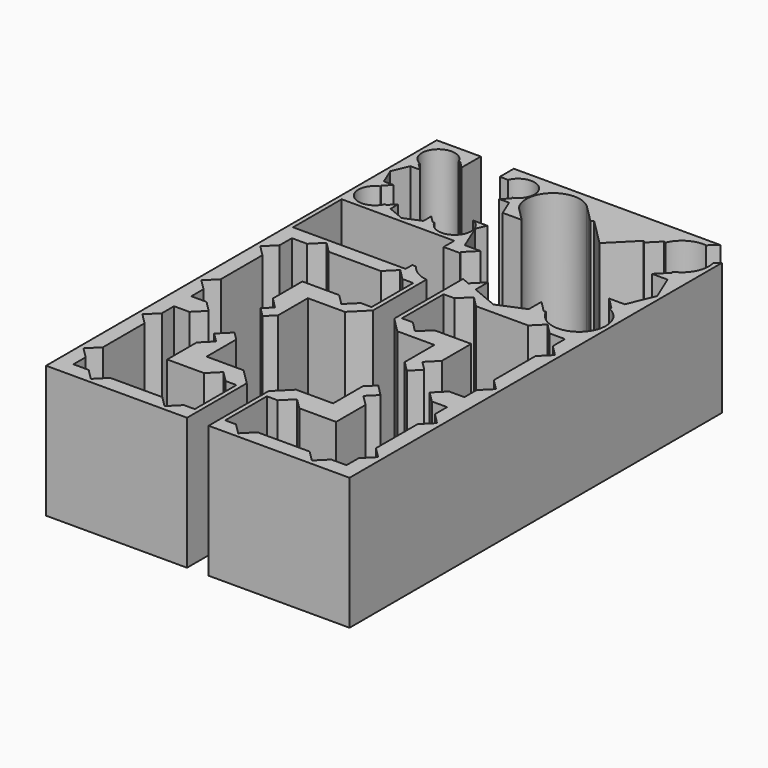
from build123d import *

# Parameters (mm, degrees)
F1_DEPTH = 4499.991


# Not quite as in the source:
# - ends of sketch curves that miss each other by under 0.0002 mm in the source are joined


with BuildPart() as f1:
    # F0 (on Top) → F1 (new body)
    with BuildSketch(Plane.XY):
        with BuildLine():
            Line((11073.483338, 6645.118502), (11073.483338, 4872.327475))
            Line((11073.483338, 4872.327475), (15876.504585, 4872.327475))
            Line((15876.504585, 4872.327475), (15876.504585, 17254.221114))
            Line((15876.504585, 17254.221114), (15876.504585, 19076.558289))
            Line((15876.504585, 19076.558289), (15876.504585, 20733.621973))
            Line((15876.504585, 20733.621973), (15702.275692, 20580.208536))
            ThreePointArc((15702.275692, 20580.208536), (15633.5838339576, 19946.0126227225), (15166.584054889, 19511.4620112681))
            Line((15166.584054889, 19511.4620112681), (15191.756497, 19450.687045))
            Line((15191.756497, 19450.687045), (14818.513126, 19076.558289))
            Line((14818.513126, 19076.558289), (15346.717243, 19076.558289))
            Line((15346.717243, 19076.558289), (15347.514333, 19076.558289))
            Line((15347.514333, 19076.558289), (15726.512005, 18166.38871))
            Line((15726.512005, 18166.38871), (15349.006362, 17254.221114))
            Line((15349.006362, 17254.221114), (14819.1259, 17254.221114))
            Line((14819.1259, 17254.221114), (15194.500704, 16873.268429))
            Line((15194.500704, 16873.268429), (15170.853649, 16814.093734))
            ThreePointArc((15170.853649, 16814.093734), (15468.5250886788, 15323.8342600463), (13978.3168296804, 15621.7619852804))
            Line((13978.3168296804, 15621.7619852804), (13914.313864, 15595.390381))
            Line((13914.313864, 15595.390381), (13530.24545, 15979.458795))
            Line((13530.24545, 15979.458795), (13530.418404, 15437.211152))
            Line((13530.418404, 15437.211152), (12623.742997, 15063.627113))
            Line((12623.742997, 15063.627113), (11718.060122, 15440.753437))
            Line((11718.060122, 15440.753437), (11718.060122, 15968.750579))
            Line((11718.060122, 15968.750579), (11345.909345, 15595.717009))
            Line((11345.909345, 15595.717009), (11268.913573, 15627.114975))
            Line((11268.913573, 15627.114975), (11073.483338, 15706.809113))
            Line((11073.483338, 15706.809113), (11073.483338, 15333.955362))
            Line((11073.483338, 15333.955362), (11073.483338, 15054.703366))
            Line((11073.483338, 15054.703366), (11073.483338, 12780.422037))
            Line((11073.483338, 12780.422037), (11593.04864, 12260.856735))
            Line((11593.04864, 12260.856735), (12856.236588, 12260.856735))
            Line((12856.236588, 12260.856735), (12856.236588, 10997.668787))
            Line((12856.236588, 10997.668787), (13210.164784, 10643.740591))
            Line((13210.164784, 10643.740591), (13540.371809, 10973.947616))
            Line((13540.371809, 10973.947616), (13216.179676, 11298.139749))
            Line((13216.179676, 11298.139749), (13583.808247, 11665.768321))
            Line((13583.808247, 11665.768321), (13583.808247, 12920.930775))
            Line((13583.808247, 12920.930775), (12328.645793, 12920.930775))
            Line((12328.645793, 12920.930775), (11961.017221, 12553.302204))
            Line((11961.017221, 12553.302204), (11593.38865, 12920.930775))
            Line((11593.38865, 12920.930775), (11223.483338, 12920.930775))
            Line((11223.483338, 12920.930775), (11223.483338, 14695.998542))
            Line((11223.483338, 14695.998542), (11593.38865, 14695.998542))
            Line((11593.38865, 14695.998542), (11961.017221, 15063.627113))
            Line((11961.017221, 15063.627113), (12328.645793, 14695.998542))
            Line((12328.645793, 14695.998542), (13583.808247, 14695.998542))
            Line((13583.808247, 14695.998542), (14103.713559, 14695.998542))
            Line((14103.713559, 14695.998542), (14471.342131, 15063.627113))
            Line((14471.342131, 15063.627113), (14838.970702, 14695.998542))
            Line((14838.970702, 14695.998542), (15358.876014, 14695.998542))
            Line((15358.876014, 14695.998542), (15358.876014, 14176.09323))
            Line((15358.876014, 14176.09323), (15726.504585, 13808.464659))
            Line((15726.504585, 13808.464659), (15358.876014, 13440.836087))
            Line((15358.876014, 13440.836087), (15358.876014, 12920.930775))
            Line((15358.876014, 12920.930775), (15358.876014, 11665.768321))
            Line((15358.876014, 11665.768321), (15726.504585, 11298.139749))
            Line((15726.504585, 11298.139749), (15358.876014, 10930.511178))
            Line((15358.876014, 10930.511178), (15358.876014, 10410.605866))
            Line((15358.876014, 10410.605866), (14838.970702, 10410.605866))
            Line((14838.970702, 10410.605866), (14471.342131, 10042.977294))
            Line((14471.342131, 10042.977294), (14838.970702, 9675.348723))
            Line((14838.970702, 9675.348723), (15358.876014, 9675.348723))
            Line((15358.876014, 9675.348723), (15358.876014, 9155.443411))
            Line((15358.876014, 9155.443411), (15726.504585, 8787.81484))
            Line((15726.504585, 8787.81484), (15358.876014, 8420.186268))
            Line((15358.876014, 8420.186268), (15358.876014, 7900.280956))
            Line((15358.876014, 7900.280956), (15358.876014, 6645.118502))
            Line((15358.876014, 6645.118502), (15726.504585, 6277.48993))
            Line((15726.504585, 6277.48993), (15358.876014, 5909.861359))
            Line((15358.876014, 5909.861359), (15358.876014, 5389.956047))
            Line((15358.876014, 5389.956047), (14838.970702, 5389.956047))
            Line((14838.970702, 5389.956047), (14471.342131, 5022.327475))
            Line((14471.342131, 5022.327475), (14103.713559, 5389.956047))
            Line((14103.713559, 5389.956047), (13583.808247, 5389.956047))
            Line((13583.808247, 5389.956047), (12328.645793, 5389.956047))
            Line((12328.645793, 5389.956047), (11961.017221, 5022.327475))
            Line((11961.017221, 5022.327475), (11593.38865, 5389.956047))
            Line((11593.38865, 5389.956047), (11223.483338, 5389.956047))
            Line((11223.483338, 5389.956047), (11223.483338, 7165.023813))
            Line((11223.483338, 7165.023813), (11593.38865, 7165.023813))
            Line((11593.38865, 7165.023813), (11961.017221, 7532.652385))
            Line((11961.017221, 7532.652385), (12328.645793, 7165.023813))
            Line((12328.645793, 7165.023813), (13583.808247, 7165.023813))
            Line((13583.808247, 7165.023813), (13583.808247, 8420.186268))
            Line((13583.808247, 8420.186268), (13216.179676, 8787.81484))
            Line((13216.179676, 8787.81484), (13540.371809, 9112.006973))
            Line((13540.371809, 9112.006973), (13148.682055, 9503.696727))
            Line((13148.682055, 9503.696727), (12856.236588, 9211.25126))
            Line((12856.236588, 9211.25126), (12856.236588, 7948.063312))
            Line((12856.236588, 7948.063312), (11593.04864, 7948.063312))
            Line((11593.04864, 7948.063312), (11073.483338, 7428.49801))
            Line((11073.483338, 7428.49801), (11073.483338, 6645.118502))
        make_face()
    extrude(amount=F1_DEPTH)


with BuildPart() as f1b:
    # F0 (on Top) → F1, piece 2 (new body)
    with BuildSketch(Plane.XY):
        with BuildLine():
            Line((5685.204947, 6277.48993), (6052.833519, 6645.118502))
            Line((6052.833519, 6645.118502), (6052.833519, 7900.280956))
            Line((6052.833519, 7900.280956), (6052.833519, 8420.186268))
            Line((6052.833519, 8420.186268), (5685.204947, 8787.81484))
            Line((5685.204947, 8787.81484), (6052.833519, 9155.443411))
            Line((6052.833519, 9155.443411), (6052.833519, 9675.348723))
            Line((6052.833519, 9675.348723), (6572.738831, 9675.348723))
            Line((6572.738831, 9675.348723), (6940.367402, 10042.977294))
            Line((6940.367402, 10042.977294), (6572.738831, 10410.605866))
            Line((6572.738831, 10410.605866), (6052.833519, 10410.605866))
            Line((6052.833519, 10410.605866), (6052.833519, 10930.511178))
            Line((6052.833519, 10930.511178), (5685.204947, 11298.139749))
            Line((5685.204947, 11298.139749), (6052.833519, 11665.768321))
            Line((6052.833519, 11665.768321), (6052.833519, 13440.836087))
            Line((6052.833519, 13440.836087), (5685.204947, 13808.464659))
            Line((5685.204947, 13808.464659), (6052.833519, 14176.09323))
            Line((6052.833519, 14176.09323), (6052.833519, 14695.998542))
            Line((6052.833519, 14695.998542), (6572.738831, 14695.998542))
            Line((6572.738831, 14695.998542), (6940.367402, 15063.627113))
            Line((6940.367402, 15063.627113), (7307.995974, 14695.998542))
            Line((7307.995974, 14695.998542), (9083.06374, 14695.998542))
            Line((9083.06374, 14695.998542), (9450.692312, 15063.627113))
            Line((9450.692312, 15063.627113), (9818.320883, 14695.998542))
            Line((9818.320883, 14695.998542), (10188.226195, 14695.998542))
            Line((10188.226195, 14695.998542), (10188.226195, 12920.930775))
            Line((10188.226195, 12920.930775), (9818.320883, 12920.930775))
            Line((9818.320883, 12920.930775), (9450.692312, 12553.302204))
            Line((9450.692312, 12553.302204), (9083.06374, 12920.930775))
            Line((9083.06374, 12920.930775), (8563.158428, 12920.930775))
            Line((8563.158428, 12920.930775), (7827.901285, 12920.930775))
            Line((7827.901285, 12920.930775), (7827.901285, 11665.768321))
            Line((7827.901285, 11665.768321), (8195.529857, 11298.139749))
            Line((8195.529857, 11298.139749), (7922.546809, 11025.156701))
            Line((7922.546809, 11025.156701), (8246.738943, 10700.964566))
            Line((8246.738943, 10700.964566), (8543.443165, 10997.668788))
            Line((8543.443165, 10997.668788), (8543.443165, 12260.856735))
            Line((8543.443165, 12260.856735), (9806.631112, 12260.856735))
            Line((9806.631112, 12260.856735), (10338.226195, 12792.451818))
            Line((10338.226195, 12792.451818), (10338.226195, 15054.703366))
            Line((10338.226195, 15054.703366), (10338.226195, 15068.484941))
            ThreePointArc((10338.226195, 15068.484941), (9950.3897153599, 15203.9895780945), (9654.1428783757, 15488.623471252))
            Line((9654.1428783757, 15488.623471252), (9520.981409, 15488.623471))
            Line((9520.981409, 15488.623471), (9520.981409, 15204.703366))
            Line((9520.981409, 15204.703366), (5685.204947, 15204.703366))
            Line((5685.204947, 15204.703366), (5685.204947, 17276.605614))
            Line((5685.204947, 17276.605614), (9520.981409, 17276.605614))
            Line((9520.981409, 17276.605614), (9520.981409, 16821.953137))
            Line((9520.981409, 16821.953137), (10077.294221, 16821.953137))
            Line((10077.294221, 16821.953137), (10055.239687, 16875.426648))
            Line((10055.239687, 16875.426648), (10433.137727, 17254.221114))
            Line((10433.137727, 17254.221114), (9898.479631, 17254.221114))
            Line((9898.479631, 17254.221114), (9520.973988, 18166.38871))
            Line((9520.973988, 18166.38871), (9662.888697, 18507.199381))
            Line((9662.888697, 18507.199381), (9520.981409, 18507.199381))
            Line((9520.981409, 18507.199381), (9176.957393, 18507.199381))
            ThreePointArc((9176.957393, 18507.199381), (9367.7478972803, 17592.1245511956), (8451.2763102301, 17776.0886560934))
            Line((8451.2763102301, 17776.0886560934), (8400.824685, 17755.300708))
            Line((8400.824685, 17755.300708), (8163.423173, 17992.702219))
            Line((8163.423173, 17992.702219), (8163.53008, 17657.526492))
            Line((8163.53008, 17657.526492), (7603.093178, 17426.605614))
            Line((7603.093178, 17426.605614), (7043.269783, 17659.716059))
            Line((7043.269783, 17659.716059), (7043.269783, 17986.083225))
            Line((7043.269783, 17986.083225), (6813.234837, 17755.502604))
            Line((6813.234837, 17755.502604), (6764.950405, 17775.192425))
            ThreePointArc((6764.950405, 17775.192425), (5851.1057030693, 17589.8583034155), (6032.8005637983, 18504.433534489))
            Line((6032.8005637983, 18504.433534489), (6015.442265, 18546.520536))
            Line((6015.442265, 18546.520536), (6249.029726, 18780.6621))
            Line((6249.029726, 18780.6621), (5918.545272, 18780.6621))
            Line((5918.545272, 18780.6621), (5685.2049467962, 19344.4827659157))
            Line((5685.2049467962, 19344.4827659157), (5685.20036, 19344.493849))
            Line((5685.20036, 19344.493849), (5685.2049470847, 19344.5048649647))
            Line((5685.2049470847, 19344.5048649647), (5919.46753, 19907.09058))
            Line((5919.46753, 19907.09058), (6249.034812, 19907.09058))
            Line((6249.034812, 19907.09058), (6016.355837, 20139.769555))
            Line((6016.355837, 20139.769555), (6032.49935, 20179.28865))
            ThreePointArc((6032.49935, 20179.28865), (5847.1879030317, 21092.709678888), (6761.6081149333, 20912.3933349723))
            Line((6761.6081149333, 20912.3933349723), (6801.038387, 20928.7526))
            Line((6801.038387, 20928.7526), (7034.985602, 20697.348815))
            Line((7034.985602, 20697.348815), (7038.771867, 21511.85029))
            Line((7038.771867, 21511.85029), (5535.204947, 21511.85029))
            Line((5535.204947, 21511.85029), (5535.204947, 19907.09058))
            Line((5535.204947, 19907.09058), (5535.204947, 18780.6621))
            Line((5535.204947, 18780.6621), (5535.204947, 4872.327475))
            Line((5535.204947, 4872.327475), (10338.226195, 4872.327475))
            Line((10338.226195, 4872.327475), (10338.226195, 6645.118502))
            Line((10338.226195, 6645.118502), (10338.226195, 7416.46823))
            Line((10338.226195, 7416.46823), (9806.631112, 7948.063312))
            Line((9806.631112, 7948.063312), (8543.443165, 7948.063312))
            Line((8543.443165, 7948.063312), (8543.443165, 9211.25126))
            Line((8543.443165, 9211.25126), (8257.012588, 9497.681837))
            Line((8257.012588, 9497.681837), (7871.337724, 9112.006973))
            Line((7871.337724, 9112.006973), (8195.529857, 8787.81484))
            Line((8195.529857, 8787.81484), (7827.901285, 8420.186268))
            Line((7827.901285, 8420.186268), (7827.901285, 7900.280956))
            Line((7827.901285, 7900.280956), (7827.901285, 7165.023813))
            Line((7827.901285, 7165.023813), (9083.06374, 7165.023813))
            Line((9083.06374, 7165.023813), (9450.692312, 7532.652385))
            Line((9450.692312, 7532.652385), (9818.320883, 7165.023813))
            Line((9818.320883, 7165.023813), (10188.226195, 7165.023813))
            Line((10188.226195, 7165.023813), (10188.226195, 5389.956047))
            Line((10188.226195, 5389.956047), (9818.320883, 5389.956047))
            Line((9818.320883, 5389.956047), (9450.692312, 5022.327475))
            Line((9450.692312, 5022.327475), (9083.06374, 5389.956047))
            Line((9083.06374, 5389.956047), (7307.995974, 5389.956047))
            Line((7307.995974, 5389.956047), (6940.367402, 5022.327475))
            Line((6940.367402, 5022.327475), (6572.738831, 5389.956047))
            Line((6572.738831, 5389.956047), (6052.833519, 5389.956047))
            Line((6052.833519, 5389.956047), (6052.833519, 5909.861359))
            Line((6052.833519, 5909.861359), (5685.204947, 6277.48993))
        make_face()
    extrude(amount=F1_DEPTH)


with BuildPart() as f1c:
    # F0 (on Top) → F1, piece 3 (new body)
    with BuildSketch(Plane.XY):
        with BuildLine():
            Line((15200.587411, 21511.85029), (8162.455407, 21511.85029))
            Line((8162.455407, 21511.85029), (8162.455407, 21269.15029))
            Line((8162.455407, 21269.15029), (8162.455407, 20917.141588))
            Line((8162.455407, 20917.141588), (8441.297517, 20911.537516))
            ThreePointArc((8441.297517, 20911.537516), (9354.7735556948, 21093.6224814193), (9173.16841879, 20180.050928507))
            Line((9173.16841879, 20180.050928507), (9190.441328, 20138.34816))
            Line((9190.441328, 20138.34816), (8954.201085, 19901.547522))
            Line((8954.201085, 19901.547522), (9286.226126, 19907.09058))
            Line((9286.226126, 19907.09058), (9520.981409, 19340.310256))
            Line((9520.981409, 19340.310256), (10169.393989, 19340.310256))
            Line((10169.393989, 19340.310256), (9676.547811, 19833.156433))
            ThreePointArc((9676.547811, 19833.156433), (9808.1348242566, 21028.8684445278), (11010.7357948497, 21057.0333378199))
            Line((11010.7357948497, 21057.0333378199), (11337.149436, 20730.619698))
            Line((11337.149436, 20730.619698), (11633.784733, 20433.984401))
            Line((11633.784733, 20433.984401), (11704.495411, 20504.695079))
            Line((11704.495411, 20504.695079), (12621.459658, 19587.730831))
            Line((12621.459658, 19587.730831), (13457.720978, 20427.075136))
            Line((13457.720978, 20427.075136), (13528.561638, 20356.49468))
            Line((13528.561638, 20356.49468), (13903.70486, 20733.020915))
            Line((13903.70486, 20733.020915), (13973.097584, 20704.321769))
            ThreePointArc((13973.097584, 20704.321769), (14352.2418677561, 21141.4460608629), (14917.9736488687, 21263.0009288184))
            Line((14917.9736488687, 21263.0009288184), (15200.587411, 21511.85029))
        make_face()
    extrude(amount=F1_DEPTH)


solid = Compound([f1.part, f1b.part, f1c.part])
